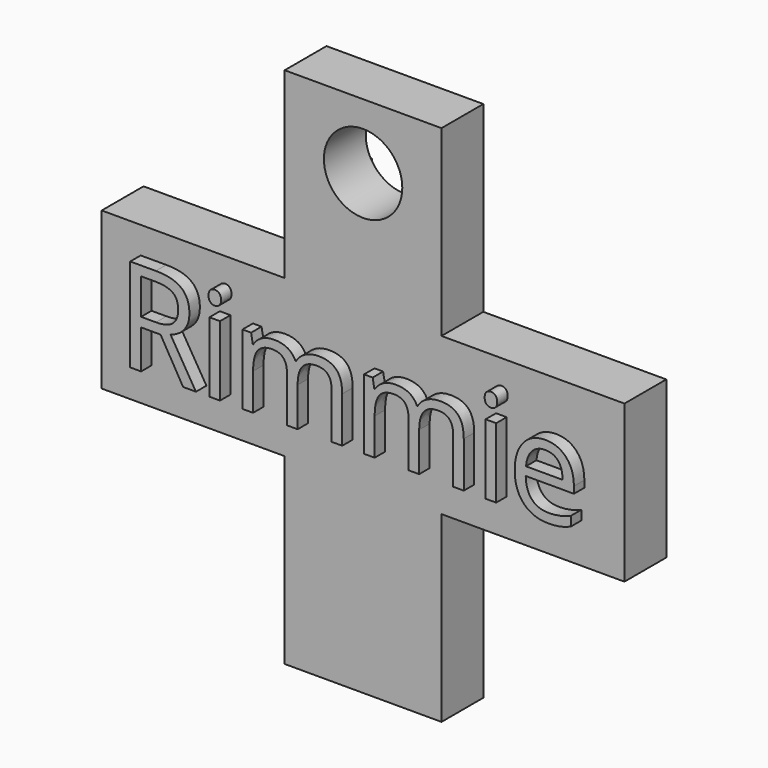
from build123d import *

# Parameters (mm, degrees)
F0_W           = 35
F0_H           = 30
F0_W_2         = 30
F0_H_2         = 35
F0_R           = 7.5
F1_DEPTH       = 10
F2_TEXT_SIZE   = 25
F3_DEPTH       = 2.5
F5_TEXT_SIZE   = 26.3601619129
F6_DEPTH       = 2.5
F7_TEXT_SIZE   = 11.4096225136
F8_DEPTH       = 2.5
F10_DEPTH      = 2.5
F4_TEXT_SIZE   = 20.8333333333
F4_TEXT_SIZE_2 = 21.2455039016
F11_DEPTH      = 2.5


# Not quite as in the source:
# - Text() gives the source's letters only with a copy of the font that has no kerning and outlines rounded to 1/6400 em; it was checked with that copy


with BuildPart() as f1:
    # F0 (on Front) → F1 (new body)
    with BuildSketch(Plane.XZ):
        with Locations((32.5, 0)):
            Rectangle(F0_W, F0_H)
        with Locations((0, -32.5)):
            Rectangle(F0_W_2, F0_H_2)
        Rectangle(F0_W_2, F0_H)
        with Locations((-32.5, 0)):
            Rectangle(F0_W, F0_H)
        with Locations((0, 32.5)):
            Rectangle(F0_W_2, F0_H_2)
        with Locations((0, 37.5)):
            Circle(F0_R, mode=Mode.SUBTRACT)
    extrude(amount=F1_DEPTH)

    # F2 (on face) → F3 (join)
    with BuildSketch(Plane.XZ.offset(10)):
        with Locations((-44.9999811153, -7.9999967776)):
            Text('Rimmie', F2_TEXT_SIZE, font='Open Sans', text_align=(TextAlign.LEFT, TextAlign.BOTTOM))
    extrude(amount=F3_DEPTH)

    # F5 (on face) → F6 (join)
    with BuildSketch(Plane(origin=(0, 0, 0), x_dir=(-1, 0, 0), z_dir=(0, 1, 0))):
        with Locations((-10.1978396997, -9.0647479519)):
            Text('&', F5_TEXT_SIZE, font='Open Sans', text_align=(TextAlign.LEFT, TextAlign.BOTTOM))
    extrude(amount=F6_DEPTH)

    # F7 (on face) → F8 (join)
    with BuildSketch(Plane(origin=(0, 0, 0), x_dir=(-1, 0, 0), z_dir=(0, 1, 0))):
        with Locations((19.2625913769, -2.8327321634)):
            Text('Miss', F7_TEXT_SIZE, font='Open Sans', text_align=(TextAlign.LEFT, TextAlign.BOTTOM))
    extrude(amount=F8_DEPTH)

    # F9 (on face) → F10 (join)
    with BuildSketch(Plane(origin=(0, 0, 0), x_dir=(-1, 0, 0), z_dir=(0, 1, 0))):
        with BuildLine():
            add(Edge.make_bspline(
                [(-32.5764380395, 7.365108002), (-29.4961095259, 9.7188709592), (-23.4467530819, 14.341349065), (-14.2254942959, 1.7775788416), (-25.739878733, -5.5587131067), (-32.5764380395, -9.9145686254)],
                knots=[0, 0, 0, 0, 0.2965122064, 0.5823106264, 1, 1, 1, 1], degree=3))
            add(Edge.make_bspline(
                [(-32.5764380395, 7.365108002), (-35.6567665532, 9.7188709592), (-41.7061229972, 14.341349065), (-50.9273817832, 1.7775788416), (-39.4129973461, -5.5587131067), (-32.5764380395, -9.9145686254)],
                knots=[0, 0, 0, 0, 0.2965122064, 0.5823106264, 1, 1, 1, 1], degree=3))
        make_face()
    extrude(amount=F10_DEPTH)

    # F4 (on face) → F11 (join)
    with BuildSketch(Plane(origin=(0, 0, 0), x_dir=(-1, 0, 0), z_dir=(0, 1, 0))):
        with Locations((6.2522479436, 17.3313878657)):
            Text('I', F4_TEXT_SIZE, font='Open Sans', text_align=(TextAlign.LEFT, TextAlign.BOTTOM))
        with Locations((-8.2149291411, -41.6411869228)):
            Text('U', F4_TEXT_SIZE_2, font='Open Sans', text_align=(TextAlign.LEFT, TextAlign.BOTTOM))
    extrude(amount=F11_DEPTH)


solid = f1.part
